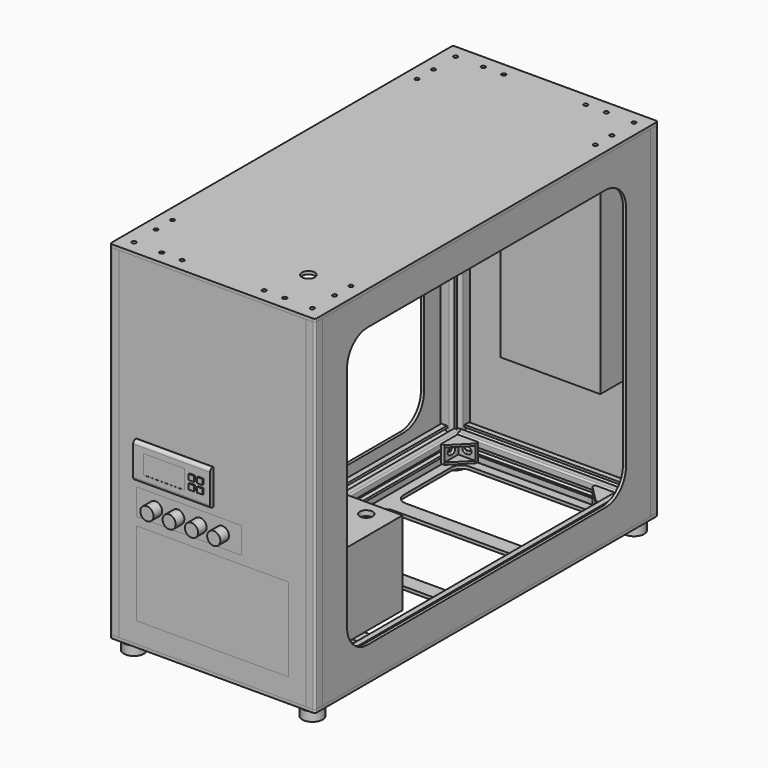
from build123d import *
from build123d import SkipClean  # not in build123d's __all__

# Parameters (mm, degrees)
F0_W           = 182
F0_H           = 332.5
F1_DEPTH       = 3
F3_DEPTH       = 332.5
F4_R           = 2
F5_W           = 400
F5_H           = 332.5
F6_DEPTH       = 3
F7_R           = 2.5
F12_DEPTH      = 380
F20_R          = 2
F21_DEPTH      = 3
F23_R          = 2
F24_DEPTH      = 2.5
F28_R          = 10
F28_R_2        = 1.6
F29_DEPTH      = 9
F34_DEPTH      = 3.001
F34_DEPTH_BACK = 197.001
F35_R          = 2.5
F36_DEPTH      = 162
F37_W          = 4
F37_H          = 3.9499961089
F38_DEPTH      = 20
F42_W          = 20
F42_H          = 17
F43_DEPTH      = 3.2
F44_W          = 3.2
F44_H          = 17
F45_DEPTH      = 16.8
F48_DEPTH      = 26.201
F50_DEPTH      = 2.1
F52_DEPTH      = 2.1
F61_DEPTH      = 3
F62_W          = 97.5
F62_H          = 198.5
F63_DEPTH      = 43.5
F64_W          = 148.5
F64_H          = 81.5
F65_DEPTH      = 3
F66_W          = 148.5
F66_H          = 81.5
F67_DEPTH      = 140
F68_W          = 102.45
F68_H          = 25.5
F68_W_2        = 70
F68_H_2        = 28.5
F69_DEPTH      = 3
F70_W          = 102.45
F70_H          = 25.5
F71_DEPTH      = 95.25
F72_W          = 70
F72_H          = 28.5
F73_DEPTH      = 82
F74_W          = 75
F74_H          = 34.45
F75_DEPTH      = 4
F76_R          = 3
F77_W          = 40
F77_H          = 18.5
F78_DEPTH      = 0.1
F79_W          = 5.25
F79_H          = 5.25
F80_DEPTH      = 1
F81_R          = 6.425
F82_DEPTH      = 10.5
F83_R          = 0.725
F84_DEPTH      = 102.45
F85_R          = 6.35
F86_DEPTH      = 5
F87_T          = 5
F88_W          = 38
F88_H          = 38
F89_DEPTH      = 5
F90_W          = 135
F90_H          = 81.5
F91_DEPTH      = 2.5
F92_W          = 135
F92_H          = 81.5
F93_DEPTH      = 1
F94_W          = 130
F94_H          = 71.5
F95_DEPTH      = 6
F96_W          = 130
F96_H          = 71.5
F97_DEPTH      = 7.5
F98_W          = 60
F98_H          = 90
F99_DEPTH      = 5
F100_R         = 4
F101_W         = 5
F101_H         = 130
F102_DEPTH     = 71.5
F103_W         = 7
F103_H         = 9
F104_DEPTH     = 5
F105_W         = 65
F105_H         = 5
F106_DEPTH     = 76.5
F108_DEPTH     = 5
F109_W         = 27.5
F109_H         = 5
F110_DEPTH     = 34
F111_R         = 6.35
F112_DEPTH     = 5
F114_DEPTH     = 6
F115_W         = 51.5
F115_H         = 53.5
F115_R         = 10
F116_DEPTH     = 6
F117_R         = 21
F118_DEPTH     = 3
F119_R         = 21
F119_R_2       = 16
F120_DEPTH     = 55
F121_R         = 33
F121_R_2       = 1.5
F121_R_3       = 16
F122_DEPTH     = 5
F123_SIZE      = 2.5
F124_R         = 1.5
F125_DEPTH     = 3
F126_R         = 6.35
F127_DEPTH     = 3
F128_W         = 194
F128_H         = 70
F128_R         = 2
F129_DEPTH     = 5


# Not quite as in the source:
# - a shell that OpenCascade refuses in one call is made with other operations: the cavity is built on its own and cut out


with BuildPart() as f1:
    # F0 (on Front) → F1 (new body)
    with BuildSketch(Plane.XZ):
        with Locations((91, 166.25)):
            Rectangle(F0_W, F0_H)
    extrude(amount=-F1_DEPTH)


with BuildPart() as f3:
    # F2 (on face) → F3 (new body, through all)
    with BuildSketch(Plane(origin=(0, 0, 0), x_dir=(1, 0, 0), z_dir=(0, 0, -1))):
        with BuildLine():
            Line((174.75, -3), (172, -3))
            Line((172, -3), (172, -11.555904481))
            ThreePointArc((172, -11.555904481), (173.608973667, -13.8917281203), (176.3648576591, -13.2209287785))
            ThreePointArc((176.3648576591, -13.2209287785), (177.2677090742, -11.5214026917), (179.166726189, -11.833273811))
            ThreePointArc((179.166726189, -11.833273811), (179.4785973083, -13.7322909258), (177.7790712215, -14.6351423409))
            ThreePointArc((177.7790712215, -14.6351423409), (177.1082718797, -17.391026333), (179.444095519, -19))
            Line((179.444095519, -19), (188, -19))
            Line((188, -19), (188, -16.25))
            Line((188, -16.25), (186.5, -16.25))
            Line((186.5, -16.25), (186.5, -17.3364773399))
            Line((186.5, -17.3364773399), (182.75, -17.3364773399))
            Line((182.75, -17.3364773399), (182.75, -16.25))
            Line((182.75, -16.25), (181, -16.25))
            Line((181, -16.25), (181, -11.75))
            Line((181, -11.75), (182.75, -11.75))
            Line((182.75, -11.75), (182.75, -10.6635226601))
            Line((182.75, -10.6635226601), (186.5, -10.6635226601))
            Line((186.5, -10.6635226601), (186.5, -11.75))
            Line((186.5, -11.75), (188, -11.75))
            Line((188, -11.75), (188, -9))
            Line((188, -9), (191, -9))
            Line((191, -9), (191, 0))
            Line((191, 0), (182, 0))
            Line((182, 0), (182, -3))
            Line((182, -3), (179.25, -3))
            Line((179.25, -3), (179.25, -4.5))
            Line((179.25, -4.5), (180.3364773399, -4.5))
            Line((180.3364773399, -4.5), (180.3364773399, -8.25))
            Line((180.3364773399, -8.25), (179.25, -8.25))
            Line((179.25, -8.25), (179.25, -10))
            Line((179.25, -10), (174.75, -10))
            Line((174.75, -10), (174.75, -8.25))
            Line((174.75, -8.25), (173.6635226601, -8.25))
            Line((173.6635226601, -8.25), (173.6635226601, -4.5))
            Line((173.6635226601, -4.5), (174.75, -4.5))
            Line((174.75, -4.5), (174.75, -3))
        make_face()
    extrude(amount=-F3_DEPTH)

    # F4
    f4_edges = [f3.edges().sort_by_distance(p)[0] for p in [
        (191, 0, 166.25),
    ]]
    fillet(f4_edges, radius=F4_R)


with BuildPart() as f6:
    # F5 (on face) → F6 (new body)
    with BuildSketch(Plane.YZ.offset(188)):
        with Locations((209, 166.25)):
            Rectangle(F5_W, F5_H)
    extrude(amount=F6_DEPTH)


with BuildPart() as f11_1:
    # F11: instance of F3
    add(f3.part.mirror(Plane(origin=(189.5, 209, 166.25), x_dir=(1, 0, 0), z_dir=(0, -1, 0))), clean=False)


with BuildPart() as f12:
    # F7 (on face) → F12 (new body, through all)
    with BuildSketch(Plane(origin=(0, 19, 0), x_dir=(-1, 0, 0), z_dir=(0, 1, 0))):
        with BuildLine():
            ThreePointArc((-188, 1.5), (-187.5606601718, 0.4393398282), (-186.5, 0))
            Line((-186.5, 0), (-181.6000077823, 0))
            Line((-181.6000077823, 0), (-181.1, 1.8))
            Line((-181.1, 1.8), (-183.5, 1.8))
            Line((-183.5, 1.8), (-183.5, 3.4393398282))
            Line((-183.5, 3.4393398282), (-180.8393398282, 6.1))
            Line((-180.8393398282, 6.1), (-175.1606601718, 6.1))
            Line((-175.1606601718, 6.1), (-172.5, 3.4393398282))
            Line((-172.5, 3.4393398282), (-172.5, 1.8))
            Line((-172.5, 1.8), (-174.9, 1.8))
            Line((-174.9, 1.8), (-174.4000077823, 0))
            Line((-174.4000077823, 0), (-169.5, 0))
            ThreePointArc((-169.5, 0), (-168.4393398282, 0.4393398282), (-168, 1.5))
            Line((-168, 1.5), (-168, 6.3999855578))
            Line((-168, 6.3999855578), (-169.8, 6.8999764316))
            Line((-169.8, 6.8999764316), (-169.8, 4.5))
            Line((-169.8, 4.5), (-171.4393398282, 4.5))
            Line((-171.4393398282, 4.5), (-174.1, 7.1606601718))
            Line((-174.1, 7.1606601718), (-174.1, 12.8393398282))
            Line((-174.1, 12.8393398282), (-171.4393398282, 15.5))
            Line((-171.4393398282, 15.5), (-169.8, 15.5))
            Line((-169.8, 15.5), (-169.8, 13.0999764316))
            Line((-169.8, 13.0999764316), (-168, 13.5999855578))
            Line((-168, 13.5999855578), (-168, 18.5))
            ThreePointArc((-168, 18.5), (-168.4393398282, 19.5606601718), (-169.5, 20))
            Line((-169.5, 20), (-174.3999922177, 20))
            Line((-174.3999922177, 20), (-174.9, 18.2))
            Line((-174.9, 18.2), (-172.5, 18.2))
            Line((-172.5, 18.2), (-172.5, 16.5606601718))
            Line((-172.5, 16.5606601718), (-175.1606601718, 13.9))
            Line((-175.1606601718, 13.9), (-180.8393398282, 13.9))
            Line((-180.8393398282, 13.9), (-183.5, 16.5606601718))
            Line((-183.5, 16.5606601718), (-183.5, 18.2))
            Line((-183.5, 18.2), (-181.1, 18.2))
            Line((-181.1, 18.2), (-181.5999922177, 20))
            Line((-181.5999922177, 20), (-186.5, 20))
            ThreePointArc((-186.5, 20), (-187.5606601718, 19.5606601718), (-188, 18.5))
            Line((-188, 18.5), (-188, 13.6000144422))
            Line((-188, 13.6000144422), (-186.2, 13.1000235684))
            Line((-186.2, 13.1000235684), (-186.2, 15.5))
            Line((-186.2, 15.5), (-184.5606601718, 15.5))
            Line((-184.5606601718, 15.5), (-181.9, 12.8393398282))
            Line((-181.9, 12.8393398282), (-181.9, 7.1606601718))
            Line((-181.9, 7.1606601718), (-184.5606601718, 4.5))
            Line((-184.5606601718, 4.5), (-186.2, 4.5))
            Line((-186.2, 4.5), (-186.2, 6.9000235684))
            Line((-186.2, 6.9000235684), (-188, 6.4000144422))
            Line((-188, 6.4000144422), (-188, 1.5))
        make_face()
        with Locations((-178, 10)):
            Circle(F7_R, mode=Mode.SUBTRACT)
    extrude(amount=F12_DEPTH)


with BuildPart() as f13_1:
    # F13: instance of F3
    add(f3.part.mirror(Plane(origin=(91, 1.5, 166.25), x_dir=(0, 1, 0), z_dir=(1, 0, 0))), clean=False)


with BuildPart() as f14_1:
    # F14: instance of F11_1
    add(f11_1.part.mirror(Plane(origin=(91, 1.5, 166.25), x_dir=(0, 1, 0), z_dir=(1, 0, 0))), clean=False)


with BuildPart() as f15_1:
    # F15: instance of F6
    add(f6.part.mirror(Plane(origin=(91, 1.5, 166.25), x_dir=(0, 1, 0), z_dir=(1, 0, 0))), clean=False)


with BuildPart() as f16_1:
    # F16: instance of F12
    add(f12.part.mirror(Plane(origin=(91, 1.5, 166.25), x_dir=(0, 1, 0), z_dir=(1, 0, 0))), clean=False)


with BuildPart() as f17_1:
    # F17: instance of F12
    add(f12.part.mirror(Plane(origin=(91, 1.5, 166.25), x_dir=(1, 0, 0), z_dir=(0, 0, 1))), clean=False)


with BuildPart() as f18_1:
    # F18: instance of F16_1
    add(f16_1.part.mirror(Plane(origin=(91, 1.5, 166.25), x_dir=(1, 0, 0), z_dir=(0, 0, 1))), clean=False)


with BuildPart() as f19_1:
    # F19: instance of F1
    add(f1.part.mirror(Plane(origin=(189.5, 209, 166.25), x_dir=(1, 0, 0), z_dir=(0, -1, 0))), clean=False)

    # F117 (on face) → F118 (cut, through all)
    with BuildSketch(Plane.XZ.offset(-415)):
        with Locations((42.25, 291.075)):
            Circle(F117_R)
    extrude(amount=-F118_DEPTH, mode=Mode.SUBTRACT)

    # F124 (on face) → F125 (cut, through all)
    with BuildSketch(Plane(origin=(0, 418, 0), x_dir=(-1, 0, 0), z_dir=(0, 1, 0))):
        with Locations((-42.25, 318.075)):
            Circle(F124_R)
        with Locations((-23.158116908, 310.166883092)):
            Circle(F124_R)
        with Locations((-15.25, 291.075)):
            Circle(F124_R)
        with Locations((-23.158116908, 271.9831169079)):
            Circle(F124_R)
        with Locations((-42.25, 264.075)):
            Circle(F124_R)
        with Locations((-61.341883092, 271.9831169079)):
            Circle(F124_R)
        with Locations((-69.25, 291.075)):
            Circle(F124_R)
        with Locations((-61.341883092, 310.166883092)):
            Circle(F124_R)
    extrude(amount=-F125_DEPTH, mode=Mode.SUBTRACT)


with BuildPart() as f21:
    # F20 (on face) → F21 (new body)
    with BuildSketch(Plane.XY.offset(332.5)):
        with BuildLine():
            ThreePointArc((-9, 2), (-8.4142135624, 0.5857864376), (-7, 0))
            Line((-7, 0), (189, 0))
            ThreePointArc((189, 0), (190.4142135624, 0.5857864376), (191, 2))
            Line((191, 2), (191, 416))
            ThreePointArc((191, 416), (190.4142135624, 417.4142135624), (189, 418))
            Line((189, 418), (-7, 418))
            ThreePointArc((-7, 418), (-8.4142135624, 417.4142135624), (-9, 416))
            Line((-9, 416), (-9, 2))
        make_face()
        with Locations((3.9999999998, 13)):
            Circle(F20_R, mode=Mode.SUBTRACT)
        with Locations((3.9999999998, 40)):
            Circle(F20_R, mode=Mode.SUBTRACT)
        with Locations((30.9999999998, 13)):
            Circle(F20_R, mode=Mode.SUBTRACT)
        with Locations((3.9999999998, 60)):
            Circle(F20_R, mode=Mode.SUBTRACT)
        with Locations((50.9999999998, 13)):
            Circle(F20_R, mode=Mode.SUBTRACT)
        with Locations((131, 13)):
            Circle(F20_R, mode=Mode.SUBTRACT)
        with Locations((151, 13)):
            Circle(F20_R, mode=Mode.SUBTRACT)
        with Locations((178, 13)):
            Circle(F20_R, mode=Mode.SUBTRACT)
        with Locations((178, 40)):
            Circle(F20_R, mode=Mode.SUBTRACT)
        with Locations((178, 60)):
            Circle(F20_R, mode=Mode.SUBTRACT)
        with Locations((3.9999999998, 358)):
            Circle(F20_R, mode=Mode.SUBTRACT)
        with Locations((3.9999999998, 378)):
            Circle(F20_R, mode=Mode.SUBTRACT)
        with Locations((3.9999999998, 405)):
            Circle(F20_R, mode=Mode.SUBTRACT)
        with Locations((30.9999999998, 405)):
            Circle(F20_R, mode=Mode.SUBTRACT)
        with Locations((50.9999999998, 405)):
            Circle(F20_R, mode=Mode.SUBTRACT)
        with Locations((131, 405)):
            Circle(F20_R, mode=Mode.SUBTRACT)
        with Locations((178, 358)):
            Circle(F20_R, mode=Mode.SUBTRACT)
        with Locations((151, 405)):
            Circle(F20_R, mode=Mode.SUBTRACT)
        with Locations((178, 378)):
            Circle(F20_R, mode=Mode.SUBTRACT)
        with Locations((178, 405)):
            Circle(F20_R, mode=Mode.SUBTRACT)
    extrude(amount=F21_DEPTH)


with BuildPart() as f22_1:
    # F22: instance of F21
    add(f21.part.mirror(Plane(origin=(91, 1.5, 166.25), x_dir=(1, 0, 0), z_dir=(0, 0, 1))), clean=False)

    # F60 (on face) → F61 (cut)
    with BuildSketch(Plane(origin=(0, 0, -3), x_dir=(1, 0, 0), z_dir=(0, 0, -1))):
        with BuildLine():
            Line((150, -31), (32, -31))
            ThreePointArc((32, -31), (24.9289321881, -33.9289321881), (22, -41))
            Line((22, -41), (22, -98.75))
            ThreePointArc((22, -98.75), (24.9289321881, -105.8210678119), (32, -108.75))
            Line((32, -108.75), (150, -108.75))
            ThreePointArc((150, -108.75), (157.0710678119, -105.8210678119), (160, -98.75))
            Line((160, -98.75), (160, -41))
            ThreePointArc((160, -41), (157.0710678119, -33.9289321881), (150, -31))
        make_face()
        with BuildLine():
            ThreePointArc((22, -377), (24.9289321881, -384.0710678119), (32, -387))
            Line((32, -387), (150, -387))
            ThreePointArc((150, -387), (157.0710678119, -384.0710678119), (160, -377))
            Line((160, -377), (160, -319.25))
            ThreePointArc((160, -319.25), (157.0710678119, -312.1789321881), (150, -309.25))
            Line((150, -309.25), (32, -309.25))
            ThreePointArc((32, -309.25), (24.9289321881, -312.1789321881), (22, -319.25))
            Line((22, -319.25), (22, -377))
        make_face()
        with BuildLine():
            Line((22, -133.75), (22, -191.5))
            ThreePointArc((22, -191.5), (24.9289321881, -198.5710678119), (32, -201.5))
            Line((32, -201.5), (150, -201.5))
            ThreePointArc((150, -201.5), (157.0710678119, -198.5710678119), (160, -191.5))
            Line((160, -191.5), (160, -133.75))
            ThreePointArc((160, -133.75), (157.0710678119, -126.6789321881), (150, -123.75))
            Line((150, -123.75), (32, -123.75))
            ThreePointArc((32, -123.75), (24.9289321881, -126.6789321881), (22, -133.75))
        make_face()
        with BuildLine():
            Line((160, -284.25), (160, -226.5))
            ThreePointArc((160, -226.5), (157.0710678119, -219.4289321881), (150, -216.5))
            Line((150, -216.5), (32, -216.5))
            ThreePointArc((32, -216.5), (24.9289321881, -219.4289321881), (22, -226.5))
            Line((22, -226.5), (22, -284.25))
            ThreePointArc((22, -284.25), (24.9289321881, -291.3210678119), (32, -294.25))
            Line((32, -294.25), (150, -294.25))
            ThreePointArc((150, -294.25), (157.0710678119, -291.3210678119), (160, -284.25))
        make_face()
    extrude(amount=-F61_DEPTH, mode=Mode.SUBTRACT)


with BuildPart() as f24:
    # F23 (on face) → F24 (new body)
    with BuildSketch(Plane(origin=(0, 0, -3), x_dir=(1, 0, 0), z_dir=(0, 0, -1))):
        Polygon((186, -5), (121, -5), (121, -21), (170, -21), (170, -70), (186, -70), (186, -21), align=None)
        with Locations((178, -60)):
            Circle(F23_R, mode=Mode.SUBTRACT)
        with Locations((178, -40)):
            Circle(F23_R, mode=Mode.SUBTRACT)
        with Locations((131, -13)):
            Circle(F23_R, mode=Mode.SUBTRACT)
        with Locations((151, -13)):
            Circle(F23_R, mode=Mode.SUBTRACT)
        with Locations((178, -13)):
            Circle(F23_R, mode=Mode.SUBTRACT)
    extrude(amount=F24_DEPTH)


with BuildPart() as f25_1:
    # F25: instance of F24
    add(f24.part.mirror(Plane(origin=(91, 1.5, 166.25), x_dir=(0, 1, 0), z_dir=(1, 0, 0))), clean=False)


with BuildPart() as f26_1:
    # F26: instance of F24
    add(f24.part.mirror(Plane(origin=(189.5, 209, 166.25), x_dir=(1, 0, 0), z_dir=(0, -1, 0))), clean=False)


with BuildPart() as f27_1:
    # F27: instance of F26_1
    add(f26_1.part.mirror(Plane(origin=(91, 1.5, 166.25), x_dir=(0, 1, 0), z_dir=(1, 0, 0))), clean=False)


with BuildPart() as f29:
    # F28 (on face) → F29 (new body)
    with BuildSketch(Plane(origin=(0, 0, -5.5), x_dir=(1, 0, 0), z_dir=(0, 0, -1))):
        with Locations((178, -13)):
            Circle(F28_R)
        with Locations((178, -13)):
            Circle(F28_R_2, mode=Mode.SUBTRACT)
    extrude(amount=F29_DEPTH)


with BuildPart() as f30_1:
    # F30: instance of F29
    add(f29.part.mirror(Plane(origin=(189.5, 209, 166.25), x_dir=(1, 0, 0), z_dir=(0, -1, 0))), clean=False)


with BuildPart() as f31_1:
    # F31: instance of F29
    add(f29.part.mirror(Plane(origin=(91, 1.5, 166.25), x_dir=(0, 1, 0), z_dir=(1, 0, 0))), clean=False)


with BuildPart() as f33_1:
    # F33: instance of F30_1
    add(f30_1.part.mirror(Plane(origin=(91, 1.5, 166.25), x_dir=(0, 1, 0), z_dir=(1, 0, 0))), clean=False)


with BuildPart() as f34_tool:
    # F32 (on face) → F34 (new body, two sides)
    with BuildSketch(Plane.YZ.offset(188)) as f34_sk:
        with BuildLine():
            Line((354, 302.5), (64, 302.5))
            ThreePointArc((64, 302.5), (46.3223304703, 295.1776695297), (39, 277.5))
            Line((39, 277.5), (39, 55))
            ThreePointArc((39, 55), (46.3223304703, 37.3223304703), (64, 30))
            Line((64, 30), (354, 30))
            ThreePointArc((354, 30), (371.6776695297, 37.3223304703), (379, 55))
            Line((379, 55), (379, 277.5))
            ThreePointArc((379, 277.5), (371.6776695297, 295.1776695297), (354, 302.5))
        make_face()
    extrude(amount=F34_DEPTH)
    extrude(f34_sk.sketch, amount=-F34_DEPTH_BACK)


with BuildPart() as f6_1:
    add(f6.part, clean=False)

    # F34: cut by f34_tool
    add(f34_tool.part, mode=Mode.SUBTRACT)


with BuildPart() as f15_1_1:
    add(f15_1.part, clean=False)

    # F34: cut by f34_tool
    add(f34_tool.part, mode=Mode.SUBTRACT)


with BuildPart() as f36:
    # F35 (on face) → F36 (new body, through all)
    with BuildSketch(Plane.YZ.offset(10)):
        with BuildLine():
            ThreePointArc((3, 314), (3.4393398282, 312.9393398282), (4.5, 312.5))
            Line((4.5, 312.5), (9.3999922177, 312.5))
            Line((9.3999922177, 312.5), (9.9, 314.3))
            Line((9.9, 314.3), (7.5, 314.3))
            Line((7.5, 314.3), (7.5, 315.9393398282))
            Line((7.5, 315.9393398282), (10.1606601718, 318.6))
            Line((10.1606601718, 318.6), (15.8393398282, 318.6))
            Line((15.8393398282, 318.6), (18.5, 315.9393398282))
            Line((18.5, 315.9393398282), (18.5, 314.3))
            Line((18.5, 314.3), (16.1, 314.3))
            Line((16.1, 314.3), (16.5999922177, 312.5))
            Line((16.5999922177, 312.5), (21.5, 312.5))
            ThreePointArc((21.5, 312.5), (22.5606601718, 312.9393398282), (23, 314))
            Line((23, 314), (23, 318.9000496462))
            Line((23, 318.9000496462), (21.2, 319.4000394253))
            Line((21.2, 319.4000394253), (21.2, 317.0000002463))
            Line((21.2, 317.0000002463), (19.5606601718, 317.0000002463))
            Line((19.5606601718, 317.0000002463), (16.9000001232, 319.6606602949))
            Line((16.9000001232, 319.6606602949), (16.9000001232, 325.3393399514))
            Line((16.9000001232, 325.3393399514), (19.5606601718, 328))
            Line((19.5606601718, 328), (21.2, 328))
            Line((21.2, 328), (21.2, 325.6000394253))
            Line((21.2, 325.6000394253), (23, 326.1000496462))
            Line((23, 326.1000496462), (23, 331))
            ThreePointArc((23, 331), (22.5606601718, 332.0606601718), (21.5, 332.5))
            Line((21.5, 332.5), (16.6000077823, 332.5))
            Line((16.6000077823, 332.5), (16.1, 330.7))
            Line((16.1, 330.7), (18.5, 330.7))
            Line((18.5, 330.7), (18.5, 329.0606601718))
            Line((18.5, 329.0606601718), (15.8393398282, 326.4))
            Line((15.8393398282, 326.4), (10.1606601718, 326.4))
            Line((10.1606601718, 326.4), (7.5, 329.0606601718))
            Line((7.5, 329.0606601718), (7.5, 330.7))
            Line((7.5, 330.7), (9.9, 330.7))
            Line((9.9, 330.7), (9.4000077823, 332.5))
            Line((9.4000077823, 332.5), (4.5, 332.5))
            ThreePointArc((4.5, 332.5), (3.4393398282, 332.0606601718), (3, 331))
            Line((3, 331), (3, 326.0999503538))
            Line((3, 326.0999503538), (4.8, 325.5999605747))
            Line((4.8, 325.5999605747), (4.8, 328))
            Line((4.8, 328), (6.4393398282, 328))
            Line((6.4393398282, 328), (9.1, 325.3393398282))
            Line((9.1, 325.3393398282), (9.1, 319.6606601718))
            Line((9.1, 319.6606601718), (6.4393398282, 317))
            Line((6.4393398282, 317), (4.8, 317))
            Line((4.8, 317), (4.8, 319.3999605746))
            Line((4.8, 319.3999605746), (3, 318.8999503538))
            Line((3, 318.8999503538), (3, 314))
        make_face()
        with Locations((13, 322.5)):
            Circle(F35_R, mode=Mode.SUBTRACT)
    extrude(amount=F36_DEPTH)

    # F37 (on face) → F38 (cut)
    with BuildSketch(Plane.XY.offset(332.5)):
        with Locations((12, 21.0250019456)):
            Rectangle(F37_W, F37_H)
        with Locations((170, 21.0250019456)):
            Rectangle(F37_W, F37_H)
    extrude(amount=-F38_DEPTH, mode=Mode.SUBTRACT)


with BuildPart() as f39_1:
    # F39: instance of F36
    add(f36.part.mirror(Plane(origin=(189.5, 209, 166.25), x_dir=(1, 0, 0), z_dir=(0, -1, 0))), clean=False)


with BuildPart() as f40_1:
    # F40: instance of F36
    add(f36.part.mirror(Plane(origin=(91, 1.5, 166.25), x_dir=(1, 0, 0), z_dir=(0, 0, 1))), clean=False)


with BuildPart() as f41_1:
    # F41: instance of F39_1
    add(f39_1.part.mirror(Plane(origin=(91, 1.5, 166.25), x_dir=(1, 0, 0), z_dir=(0, 0, 1))), clean=False)


with BuildPart() as f43:
    # F42 (on face) → F43 (new body)
    with BuildSketch(Plane(origin=(0, 23, 0), x_dir=(-1, 0, 0), z_dir=(0, 1, 0))):
        with Locations((-24, 322.5)):
            Rectangle(F42_W, F42_H)
        with BuildLine():
            ThreePointArc((-26.85, 319.25), (-30.1, 322.5), (-26.85, 325.75))
            Line((-26.85, 325.75), (-24.35, 325.75))
            ThreePointArc((-24.35, 325.75), (-21.1, 322.5), (-24.35, 319.25))
            Line((-24.35, 319.25), (-26.85, 319.25))
        make_face(mode=Mode.SUBTRACT)
    extrude(amount=F43_DEPTH)

    # F44 (on face) → F45 (join)
    with BuildSketch(Plane(origin=(0, 26.2, 0), x_dir=(-1, 0, 0), z_dir=(0, 1, 0))):
        with Locations((-15.6, 322.5)):
            Rectangle(F44_W, F44_H)
    extrude(amount=F45_DEPTH)

    # F46: union 

    # F47 (on face) → F48 (cut, through all)
    with BuildSketch(Plane.YZ.offset(17.2)):
        with BuildLine():
            ThreePointArc((33.35, 325.75), (30.1, 322.5), (33.35, 319.25))
            Line((33.35, 319.25), (35.85, 319.25))
            ThreePointArc((35.85, 319.25), (39.1, 322.5), (35.85, 325.75))
            Line((35.85, 325.75), (33.35, 325.75))
        make_face()
    extrude(amount=-F48_DEPTH, mode=Mode.SUBTRACT)

    # F49 (on face) → F50 (join)
    with BuildSketch(Plane.XY.offset(331)):
        Polygon((17.2, 26.2), (34, 26.2), (17.2, 43), align=None)
    extrude(amount=-F50_DEPTH)

    # F51 (on face) → F52 (join)
    with BuildSketch(Plane(origin=(0, 0, 314), x_dir=(1, 0, 0), z_dir=(0, 0, -1))):
        Polygon((17.2, -43), (34, -26.2), (17.2, -26.2), align=None)
    extrude(amount=-F52_DEPTH)


with BuildPart() as f53_1:
    # F53: instance of F43
    add(f43.part.mirror(Plane(origin=(91, 1.5, 166.25), x_dir=(0, 1, 0), z_dir=(1, 0, 0))), clean=False)


with BuildPart() as f54_1:
    # F54: instance of F43
    add(f43.part.mirror(Plane(origin=(189.5, 209, 166.25), x_dir=(1, 0, 0), z_dir=(0, -1, 0))), clean=False)


with BuildPart() as f55_1:
    # F55: instance of F53_1
    add(f53_1.part.mirror(Plane(origin=(189.5, 209, 166.25), x_dir=(1, 0, 0), z_dir=(0, -1, 0))), clean=False)


with BuildPart() as f56_1:
    # F56: instance of F43
    add(f43.part.mirror(Plane(origin=(91, 1.5, 166.25), x_dir=(1, 0, 0), z_dir=(0, 0, 1))), clean=False)


with BuildPart() as f57_1:
    # F57: instance of F53_1
    add(f53_1.part.mirror(Plane(origin=(91, 1.5, 166.25), x_dir=(1, 0, 0), z_dir=(0, 0, 1))), clean=False)


with BuildPart() as f58_1:
    # F58: instance of F54_1
    add(f54_1.part.mirror(Plane(origin=(91, 1.5, 166.25), x_dir=(1, 0, 0), z_dir=(0, 0, 1))), clean=False)


with BuildPart() as f59_1:
    # F59: instance of F55_1
    add(f55_1.part.mirror(Plane(origin=(91, 1.5, 166.25), x_dir=(1, 0, 0), z_dir=(0, 0, 1))), clean=False)


with BuildPart() as f63:
    # F62 (on face) → F63 (new body)
    with BuildSketch(Plane.XZ.offset(-415)):
        with Locations((123.25, 213.25)):
            Rectangle(F62_W, F62_H)
    extrude(amount=F63_DEPTH)


with BuildPart() as f1_1:
    add(f1.part, clean=False)

    # F64 (on face) → F65 (cut, through all)
    with BuildSketch(Plane(origin=(0, 3, 0), x_dir=(-1, 0, 0), z_dir=(0, 1, 0))):
        with Locations((-91, 60.75)):
            Rectangle(F64_W, F64_H)
    extrude(amount=-F65_DEPTH, mode=Mode.SUBTRACT)

    # F68 (on face) → F69 (cut, through all)
    with BuildSketch(Plane.XZ):
        with Locations((67.975, 122.25)):
            Rectangle(F68_W, F68_H)
        with Locations((54.25, 159.25)):
            Rectangle(F68_W_2, F68_H_2)
    extrude(amount=-F69_DEPTH, mode=Mode.SUBTRACT)


with BuildPart() as f67:
    # F66 (on face) → F67 (new body)
    with BuildSketch(Plane.XZ):
        with Locations((91, 60.75)):
            Rectangle(F66_W, F66_H)
    extrude(amount=-F67_DEPTH)

    # F85 (on face) → F86 (cut)
    with BuildSketch(Plane.XY.offset(101.5)):
        with Locations((130.25, 25)):
            Circle(F85_R)
        with Locations((141.25, 54)):
            Circle(F85_R)
        with Locations((141.25, 124.5)):
            Circle(F85_R)
    extrude(amount=-F86_DEPTH, mode=Mode.SUBTRACT)

    # F87: shell of thickness 5, made by hand


with BuildPart() as f71:
    # F70 (on face) → F71 (new body)
    with BuildSketch(Plane.XZ):
        with Locations((67.975, 122.25)):
            Rectangle(F70_W, F70_H)
    extrude(amount=-F71_DEPTH)

    # F81 (on face) → F82 (join)
    with BuildSketch(Plane.XZ):
        with Locations((35.35, 122.25)):
            Circle(F81_R)
        with Locations((57.1, 122.25)):
            Circle(F81_R)
        with Locations((78.85, 122.25)):
            Circle(F81_R)
        with Locations((100.6, 122.25)):
            Circle(F81_R)
    extrude(amount=F82_DEPTH)

    # F83 (on face) → F84 (cut, through all)
    with BuildSketch(Plane(origin=(16.75, 0, 0), x_dir=(0, -1, 0), z_dir=(-1, 0, 0))):
        with Locations((-83.75, 114)):
            Circle(F83_R)
        with Locations((-23.5, 114)):
            Circle(F83_R)
    extrude(amount=-F84_DEPTH, mode=Mode.SUBTRACT)


with BuildPart() as f73:
    # F72 (on face) → F73 (new body)
    with BuildSketch(Plane.XZ):
        with Locations((54.25, 159.25)):
            Rectangle(F72_W, F72_H)
    extrude(amount=-F73_DEPTH)

    # F74 (on face) → F75 (join)
    with BuildSketch(Plane.XZ):
        with Locations((54.25, 159.25)):
            Rectangle(F74_W, F74_H)
    extrude(amount=F75_DEPTH)

    # F76
    f76_edges = [f73.edges().sort_by_distance(p)[0] for p in [
        (54.25, -4, 176.475),
        (54.25, -4, 142.025),
    ]]
    fillet(f76_edges, radius=F76_R)

    # F77 (on face) → F78 (cut)
    with BuildSketch(Plane.XZ.offset(4)):
        with Locations((46.75, 159.25)):
            Rectangle(F77_W, F77_H)
    extrude(amount=-F78_DEPTH, mode=Mode.SUBTRACT)

    # F79 (on face) → F80 (join)
    with BuildSketch(Plane.XZ.offset(4)):
        with Locations((74.375, 163.375)):
            Rectangle(F79_W, F79_H)
        with Locations((82.625, 163.375)):
            Rectangle(F79_W, F79_H)
        with Locations((82.625, 155.125)):
            Rectangle(F79_W, F79_H)
        with Locations((74.375, 155.125)):
            Rectangle(F79_W, F79_H)
    extrude(amount=F80_DEPTH)


with BuildPart() as f87_core1:
    # F87_t2: copy of F67
    add(f67.part, clean=False)

    # the walls: a layer under each face that stays
    f87_faces = [f87_core1.faces().sort_by_distance(p)[0] for p in [
        (91, 70, 101.5),
        (165.25, 70, 60.75),
        (91, 0, 60.75),
        (91, 140, 60.75),
        (16.75, 70, 60.75),
        (134.9, 124.5, 99),
        (134.9, 54, 99),
        (123.9, 25, 99),
        (91, 70, 20),
    ]]
    thicken(f87_faces, amount=-F87_T, mode=Mode.SUBTRACT)


with BuildPart() as f67_1:
    add(f67.part, clean=False)

    # what is left inside the walls is the cavity
    f87_cavity = [f87_core1.part.solids().sort_by_distance(p)[0] for p in [
        (91, 91.666667, 96.45),
    ]]
    add(f87_cavity, mode=Mode.SUBTRACT)

    # F88 (on face) → F89 (cut)
    with BuildSketch(Plane(origin=(0, 140, 0), x_dir=(-1, 0, 0), z_dir=(0, 1, 0))):
        with Locations((-51.25, 55.5)):
            Rectangle(F88_W, F88_H)
    extrude(amount=-F89_DEPTH, mode=Mode.SUBTRACT)

    # F90 (on face) → F91 (cut)
    with BuildSketch(Plane(origin=(16.75, 0, 0), x_dir=(0, -1, 0), z_dir=(-1, 0, 0))):
        with Locations((-72.5, 60.75)):
            Rectangle(F90_W, F90_H)
    extrude(amount=-F91_DEPTH, mode=Mode.SUBTRACT)

    # F92 (on face) → F93 (cut)
    with BuildSketch(Plane.YZ.offset(165.25)):
        with Locations((72.5, 60.75)):
            Rectangle(F92_W, F92_H)
    extrude(amount=-F93_DEPTH, mode=Mode.SUBTRACT)

    # F94 (on face) → F95 (join)
    with BuildSketch(Plane(origin=(160.25, 0, 0), x_dir=(0, -1, 0), z_dir=(-1, 0, 0))):
        with Locations((-70, 60.75)):
            Rectangle(F94_W, F94_H)
    extrude(amount=F95_DEPTH)

    # F96 (on face) → F97 (join)
    with BuildSketch(Plane.YZ.offset(21.75)):
        with Locations((70, 60.75)):
            Rectangle(F96_W, F96_H)
    extrude(amount=F97_DEPTH)

    # F98 (on face) → F99 (cut)
    with BuildSketch(Plane.XY.offset(101.5)):
        with Locations((61.5, 90)):
            Rectangle(F98_W, F98_H)
    extrude(amount=-F99_DEPTH, mode=Mode.SUBTRACT)

    # F100
    f100_edges = [f67_1.edges().sort_by_distance(p)[0] for p in [
        (70.25, 137.5, 36.5),
        (32.25, 137.5, 36.5),
        (32.25, 137.5, 74.5),
        (70.25, 137.5, 74.5),
        (91.5, 45, 99),
        (31.5, 45, 99),
    ]]
    fillet(f100_edges, radius=F100_R)

    # F101 (on face) → F102 (join, through all)
    with BuildSketch(Plane.XY.offset(25)):
        with Locations((96.75, 70)):
            Rectangle(F101_W, F101_H)
    extrude(amount=F102_DEPTH)

    # F103 (on face) → F104 (cut)
    with BuildSketch(Plane(origin=(94.25, 0, 0), x_dir=(0, -1, 0), z_dir=(-1, 0, 0))):
        with Locations((-11, 54.5)):
            Rectangle(F103_W, F103_H)
    extrude(amount=-F104_DEPTH, mode=Mode.SUBTRACT)

    # F105 (on face) → F106 (join)
    with BuildSketch(Plane(origin=(0, 5, 0), x_dir=(-1, 0, 0), z_dir=(0, 1, 0))):
        with Locations((-61.75, 61.5)):
            Rectangle(F105_W, F105_H)
    extrude(amount=F106_DEPTH)

    # F107 (on face) → F108 (join)
    with BuildSketch(Plane(origin=(0, 81.5, 0), x_dir=(-1, 0, 0), z_dir=(0, 1, 0))):
        Polygon((-29.25, 64), (-94.25, 64), (-94.25, 25), (-71.75, 25), (-71.75, 31), (-51.75, 31), (-51.75, 25), (-29.25, 25), align=None)
    extrude(amount=-F108_DEPTH)

    # F109 (on face) → F110 (join, through all)
    with BuildSketch(Plane.XY.offset(25)):
        with Locations((80.5, 23)):
            Rectangle(F109_W, F109_H)
    extrude(amount=F110_DEPTH)

    # F111 (on face) → F112 (cut, through all)
    with BuildSketch(Plane(origin=(0, 140, 0), x_dir=(-1, 0, 0), z_dir=(0, 1, 0))):
        with Locations((-108.75, 83.5)):
            Circle(F111_R)
        with Locations((-108.75, 51.5)):
            Circle(F111_R)
    extrude(amount=-F112_DEPTH, mode=Mode.SUBTRACT)

    # F113 (on face) → F114 (join)
    with BuildSketch(Plane.XY.offset(25)):
        with BuildLine():
            Line((36.75, 135), (36.75, 81.5))
            Line((36.75, 81.5), (51.75, 81.5))
            Line((51.75, 81.5), (51.75, 107.75))
            ThreePointArc((51.75, 107.75), (61.75, 117.75), (71.75, 107.75))
            Line((71.75, 107.75), (71.75, 81.5))
            Line((71.75, 81.5), (88.25, 81.5))
            Line((88.25, 81.5), (88.25, 135))
            Line((88.25, 135), (36.75, 135))
        make_face()
    extrude(amount=F114_DEPTH)

    # F115 (on face) → F116 (join)
    with BuildSketch(Plane.XY.offset(31)):
        with Locations((62.5, 108.25)):
            Rectangle(F115_W, F115_H)
        with Locations((61.75, 107.75)):
            Circle(F115_R, mode=Mode.SUBTRACT)
    with SkipClean():  # cleaning this boolean's faces spoils the solid; the shape is the same uncleaned
        extrude(amount=F116_DEPTH)


with BuildPart() as f120:
    # F119 (on face) → F120 (new body)
    with BuildSketch(Plane(origin=(0, 418, 0), x_dir=(-1, 0, 0), z_dir=(0, 1, 0))):
        with Locations((-42.25, 291.075)):
            Circle(F119_R)
        with Locations((-42.25, 291.075)):
            Circle(F119_R_2, mode=Mode.SUBTRACT)
    extrude(amount=-F120_DEPTH)

    # F121 (on face) → F122 (join)
    with BuildSketch(Plane(origin=(0, 418, 0), x_dir=(-1, 0, 0), z_dir=(0, 1, 0))):
        with Locations((-42.25, 291.075)):
            Circle(F121_R)
        with Locations((-61.341883092, 271.9831169079)):
            Circle(F121_R_2, mode=Mode.SUBTRACT)
        with Locations((-42.25, 264.075)):
            Circle(F121_R_2, mode=Mode.SUBTRACT)
        with Locations((-23.158116908, 271.9831169079)):
            Circle(F121_R_2, mode=Mode.SUBTRACT)
        with Locations((-69.25, 291.075)):
            Circle(F121_R_2, mode=Mode.SUBTRACT)
        with Locations((-61.341883092, 310.166883092)):
            Circle(F121_R_2, mode=Mode.SUBTRACT)
        with Locations((-42.25, 291.075)):
            Circle(F121_R_3, mode=Mode.SUBTRACT)
        with Locations((-15.25, 291.075)):
            Circle(F121_R_2, mode=Mode.SUBTRACT)
        with Locations((-42.25, 318.075)):
            Circle(F121_R_2, mode=Mode.SUBTRACT)
        with Locations((-23.158116908, 310.166883092)):
            Circle(F121_R_2, mode=Mode.SUBTRACT)
    extrude(amount=F122_DEPTH)

    # F123
    f123_edges = [f120.edges().sort_by_distance(p)[0] for p in [
        (75.25, 423, 291.075),
    ]]
    chamfer(f123_edges, length=F123_SIZE)


with BuildPart() as f21_1:
    add(f21.part, clean=False)

    # F126 (on face) → F127 (cut, through all)
    with BuildSketch(Plane(origin=(0, 0, 332.5), x_dir=(1, 0, 0), z_dir=(0, 0, -1))):
        with Locations((141.25, -54)):
            Circle(F126_R)
    extrude(amount=-F127_DEPTH, mode=Mode.SUBTRACT)


with BuildPart() as f129:
    # F128 (on face) → F129 (new body)
    with BuildSketch(Plane(origin=(0, 0, 312.5), x_dir=(1, 0, 0), z_dir=(0, 0, -1))):
        with Locations((91, -326)):
            Rectangle(F128_W, F128_H)
        with Locations((4, -346.6562764645)):
            Circle(F128_R, mode=Mode.SUBTRACT)
        with Locations((178, -346.6562764645)):
            Circle(F128_R, mode=Mode.SUBTRACT)
        with Locations((4, -307.9636530876)):
            Circle(F128_R, mode=Mode.SUBTRACT)
        with Locations((178, -307.9636530876)):
            Circle(F128_R, mode=Mode.SUBTRACT)
    extrude(amount=F129_DEPTH)


solid = Compound([f3.part, f11_1.part, f12.part, f13_1.part, f14_1.part, f16_1.part, f17_1.part, f18_1.part, f19_1.part, f22_1.part, f24.part, f25_1.part, f26_1.part, f27_1.part, f29.part, f30_1.part, f31_1.part, f33_1.part, f6_1.part, f15_1_1.part, f36.part, f39_1.part, f40_1.part, f41_1.part, f43.part, f53_1.part, f54_1.part, f55_1.part, f56_1.part, f57_1.part, f58_1.part, f59_1.part, f63.part, f1_1.part, f71.part, f73.part, f67_1.part, f120.part, f21_1.part, f129.part])
